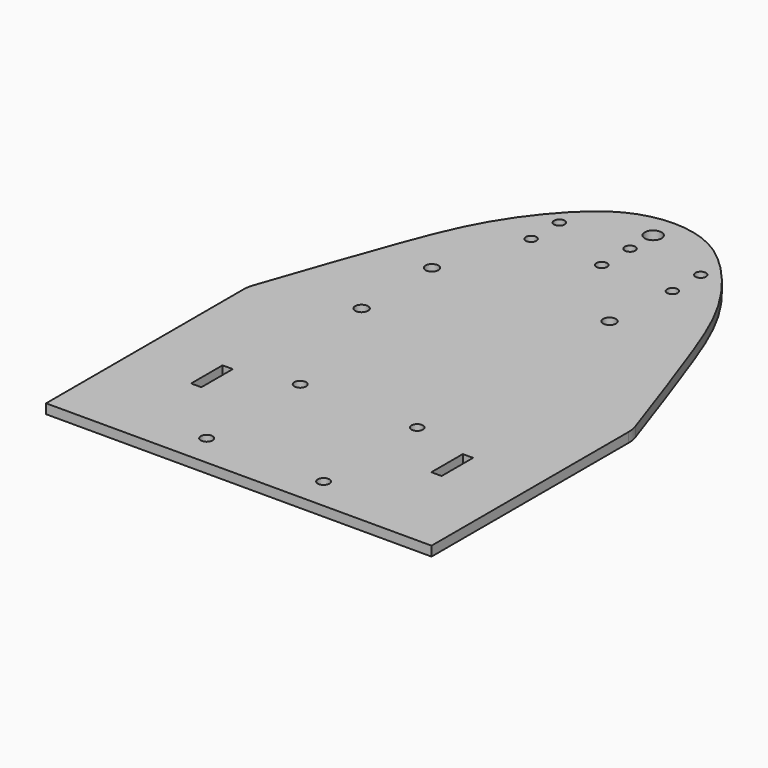
from build123d import *

# Parameters (mm, degrees)
F0_W     = 3.2
F0_H     = 12.24
F0_R     = 1.825
F0_R_2   = 2
F0_R_3   = 1.8
F0_R_4   = 1.65
F0_R_5   = 2.6
F1_DEPTH = 3


# Not quite as in the source:
# - ends of sketch curves that miss each other by under 0.0002 mm in the source are joined


with BuildPart() as f1:
    # F0 (on Top) → F1 (new body)
    with BuildSketch(Plane.XY):
        with BuildLine():
            Line((-69.459583357, 39.3533453141), (-69.459583357, -37.3673290014))
            Line((-69.459583357, -37.3673290014), (50.540416643, -37.3673290014))
            Line((50.540416643, -37.3673290014), (50.540416643, 39.3533036827))
            ThreePointArc((50.540416643, 39.3533036827), (50.404091241, 40.9988806108), (49.9988319578, 42.5995907516))
            add(Edge.make_bspline(
                [(6.5631451309, 127.1030604839), (13.1949586637, 122.5735143927), (26.4702997739, 107.0194370927), (36.3799750231, 82.2251008364), (45.1615562759, 56.6935268147), (49.9988319578, 42.5995907516)],
                knots=[0.1966855051, 0.1966855051, 0.1966855051, 0.1966855051, 0.4414351438, 0.6885909138, 0.9887974302, 0.9887974302, 0.9887974302, 0.9887974302], degree=3))
            ThreePointArc((6.5631451309, 127.1030604839), (-9.459583357, 131.9487932431), (-25.4823118448, 127.1030604839))
            add(Edge.make_bspline(
                [(-25.4823118448, 127.1030604839), (-32.1141253777, 122.5735143927), (-45.3894664879, 107.0194370927), (-55.2991588518, 82.2250580149), (-64.0807668858, 56.6933991917), (-68.9180648017, 42.5993980747)],
                knots=[0.1966855051, 0.1966855051, 0.1966855051, 0.1966855051, 0.4414351438, 0.6885909138, 0.9887987982, 0.9887987982, 0.9887987982, 0.9887987982], degree=3))
            ThreePointArc((-68.9180648017, 42.5993980747), (-69.323277955, 40.9988023559), (-69.459583357, 39.3533453141))
        make_face()
        with Locations((-46.859583357, -1.0729111145)):
            Rectangle(F0_W, F0_H, mode=Mode.SUBTRACT)
        with Locations((-27.459583357, -27.3673290014)):
            Circle(F0_R, mode=Mode.SUBTRACT)
        with Locations((-27.459583357, 9.0326709986)):
            Circle(F0_R, mode=Mode.SUBTRACT)
        with Locations((-40.759583357, 49.5270888855)):
            Circle(F0_R_2, mode=Mode.SUBTRACT)
        with Locations((8.940416643, -27.3673290014)):
            Circle(F0_R, mode=Mode.SUBTRACT)
        with Locations((8.940416643, 9.0326709986)):
            Circle(F0_R_3, mode=Mode.SUBTRACT)
        with Locations((27.940416643, -1.0729111145)):
            Rectangle(F0_W, F0_H, mode=Mode.SUBTRACT)
        with Locations((-40.759583357, 76.9270888855)):
            Circle(F0_R_2, mode=Mode.SUBTRACT)
        with Locations((-31.459583357, 103.8777989149)):
            Circle(F0_R_4, mode=Mode.SUBTRACT)
        with Locations((-9.459583357, 103.8777989149)):
            Circle(F0_R_4, mode=Mode.SUBTRACT)
        with Locations((-31.459583357, 114.8777989149)):
            Circle(F0_R_4, mode=Mode.SUBTRACT)
        with Locations((-9.459583357, 114.8777989149)):
            Circle(F0_R_4, mode=Mode.SUBTRACT)
        with Locations((-9.459583357, 123.8777989149)):
            Circle(F0_R_5, mode=Mode.SUBTRACT)
        with Locations((10.540416643, 81.9270888855)):
            Circle(F0_R_2, mode=Mode.SUBTRACT)
        with Locations((12.540416643, 103.8777989149)):
            Circle(F0_R_4, mode=Mode.SUBTRACT)
        with Locations((12.540416643, 114.8777989149)):
            Circle(F0_R_4, mode=Mode.SUBTRACT)
    extrude(amount=F1_DEPTH)


solid = f1.part
